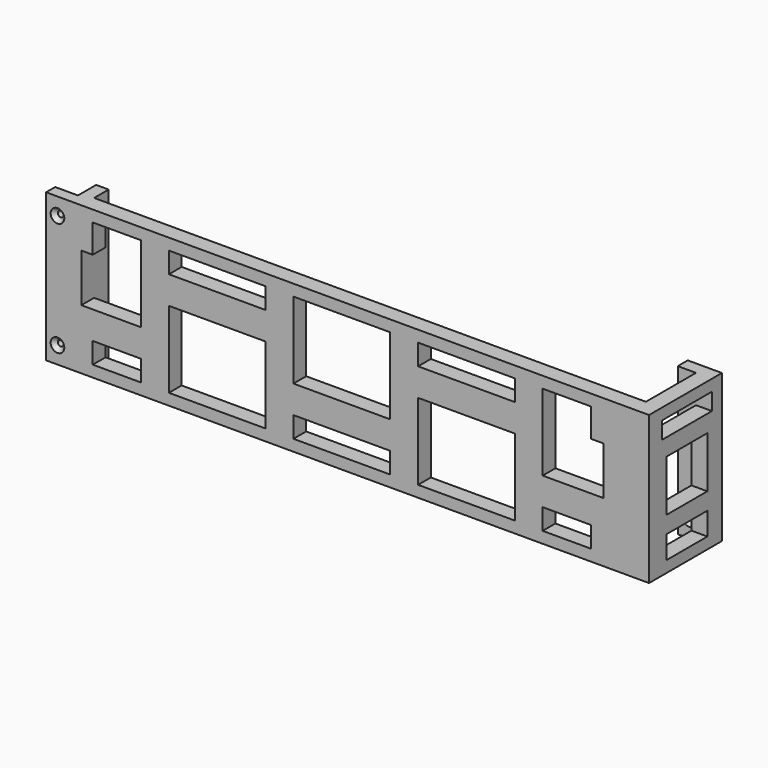
from build123d import *

# Parameters (mm, degrees)
F0_W           = 479.75
F0_H           = 130
F1_DEPTH       = 14
F2_W           = 20
F2_H           = 10
F3_DEPTH       = 130
F4_W           = 11
F4_H           = 16
F5_DEPTH       = 130
F6_W           = 42.5000000004
F6_H           = 18.3330895797
F6_W_2         = 42.5
F6_H_2         = 67.2669104207
F6_H_3         = 18.3330895795
F6_W_3         = 42.4708837634
F6_H_4         = 67.2961863439
F6_W_4         = 42.5291162366
F6_H_5         = 67.2961863442
F6_W_5         = 42.4708837635
F7_DEPTH       = 25
F8_R           = 2.5
F9_DEPTH       = 25
F10_R          = 2.5
F11_DEPTH      = 11.001
F11_DEPTH_BACK = 25
F12_R          = 2.5
F13_DEPTH      = 25
F14_SIZE       = 3.49999
F15_W          = 45
F15_H          = 20
F15_W_2        = 55
F15_H_2        = 15
F15_H_3        = 45
F16_DEPTH      = 25


# Not quite as in the source:
# - a fillet or chamfer is up to 0.001 mm smaller than in the source, because OpenCascade refuses the exact size
# - a feature names something its author has since deleted; it is built from what else it names


with BuildPart() as f1:
    # F0 (on Front) → F1 (new body)
    with BuildSketch(Plane.XZ):
        with Locations((239.875, 65)):
            Rectangle(F0_W, F0_H)
    extrude(amount=F1_DEPTH)

    # F2 (on face) → F3 (join, through all)
    with BuildSketch(Plane.XY.offset(130)):
        Polygon((479.75, 0), (479.75, -14), (509.75, -14), (509.75, 66), (479.75, 66), (479.75, 55), (495.75, 55), (495.75, 0), align=None)
        with Locations((-10, -9)):
            Rectangle(F2_W, F2_H)
    extrude(amount=-F3_DEPTH)

    # F4 (on face) → F5 (join, through all)
    with BuildSketch(Plane.XY.offset(130)):
        with Locations((5.5, 8)):
            Rectangle(F4_W, F4_H)
    extrude(amount=-F5_DEPTH)

    # F6 (on face) → F7 (cut)
    with BuildSketch(Plane.XZ.offset(14)):
        Polygon((21, 120), (21, 95), (11, 95), (11, 52.7330895796), (21, 52.7330895796), (63.5, 52.7330895796), (63.5, 120), align=None)
        with Locations((42.2499999998, 19.1665447897)):
            Rectangle(F6_W, F6_H)
        with Locations((109.15, 43.6334552101)):
            Rectangle(F6_W_2, F6_H_2)
        with Locations((151.65, 43.6334552101)):
            Rectangle(F6_W_2, F6_H_2)
        with Locations((109.15, 110.8334552102)):
            Rectangle(F6_W_2, F6_H_3)
        with Locations((151.65, 110.8334552102)):
            Rectangle(F6_W_2, F6_H_3)
        with Locations((218.5645581183, 86.351906828)):
            Rectangle(F6_W_3, F6_H_4)
        with Locations((261.0645581183, 86.351906828)):
            Rectangle(F6_W_4, F6_H_4)
        with Locations((218.5645581183, 19.1665447897)):
            Rectangle(F6_W_3, F6_H)
        with Locations((261.0645581183, 19.1665447897)):
            Rectangle(F6_W_4, F6_H)
        with Locations((328.0854418817, 43.6480931718)):
            Rectangle(F6_W_4, F6_H_5)
        with Locations((370.5854418817, 43.6480931718)):
            Rectangle(F6_W_5, F6_H_5)
        with Locations((370.5854418817, 110.8334552102)):
            Rectangle(F6_W_3, F6_H_3)
        with Locations((328.0854418817, 110.8334552102)):
            Rectangle(F6_W_4, F6_H_3)
        Polygon((458.75, 120), (416.25, 120), (416.25, 52.7330895795), (469.75, 52.7330895795), (469.75, 95), (458.75, 95), align=None)
        with Locations((437.5, 19.1665447897)):
            Rectangle(F6_W_2, F6_H)
    extrude(amount=-F7_DEPTH, mode=Mode.SUBTRACT)

    # F8 (on face) → F9 (cut)
    with BuildSketch(Plane(origin=(0, -4, 0), x_dir=(-1, 0, 0), z_dir=(0, 1, 0))):
        with Locations((10, 115)):
            Circle(F8_R)
        with Locations((10, 15)):
            Circle(F8_R)
    extrude(amount=-F9_DEPTH, mode=Mode.SUBTRACT)

    # F10 (on face) → F11 (cut, two sides)
    with BuildSketch(Plane.XZ.offset(-55)) as f11_sk:
        with Locations((489.75, 15)):
            Circle(F10_R)
        with Locations((489.75, 115)):
            Circle(F10_R)
    extrude(amount=-F11_DEPTH, mode=Mode.SUBTRACT)
    extrude(f11_sk.sketch, amount=F11_DEPTH_BACK, mode=Mode.SUBTRACT)

    # F12 (on face) → F13 (cut)
    with BuildSketch(Plane(origin=(0, 0, 0), x_dir=(0, -1, 0), z_dir=(-1, 0, 0))):
        with Locations((-6, 15)):
            Circle(F12_R)
        with Locations((-6, 115)):
            Circle(F12_R)
    extrude(amount=-F13_DEPTH, mode=Mode.SUBTRACT)

    # F14 (size 3.5 in the source; OpenCascade refuses exactly that, so slightly less here)
    f14_edges = [f1.edges().sort_by_distance(p)[0] for p in [
        (487.25, 55, 15),
        (487.25, 55, 115),
        (-7.5, -14, 15),
        (-7.5, -14, 115),
        (11, 8.5, 15),
        (11, 8.5, 115),
    ]]
    chamfer(f14_edges, length=F14_SIZE)

    # F15 (on face) → F16 (cut)
    with BuildSketch(Plane.YZ.offset(509.75)):
        with Locations((27.5, 20)):
            Rectangle(F15_W, F15_H)
        with Locations((27.5, 112.5)):
            Rectangle(F15_W_2, F15_H_2)
        with Locations((27.5, 67.5)):
            Rectangle(F15_W, F15_H_3)
    extrude(amount=-F16_DEPTH, mode=Mode.SUBTRACT)


solid = f1.part
